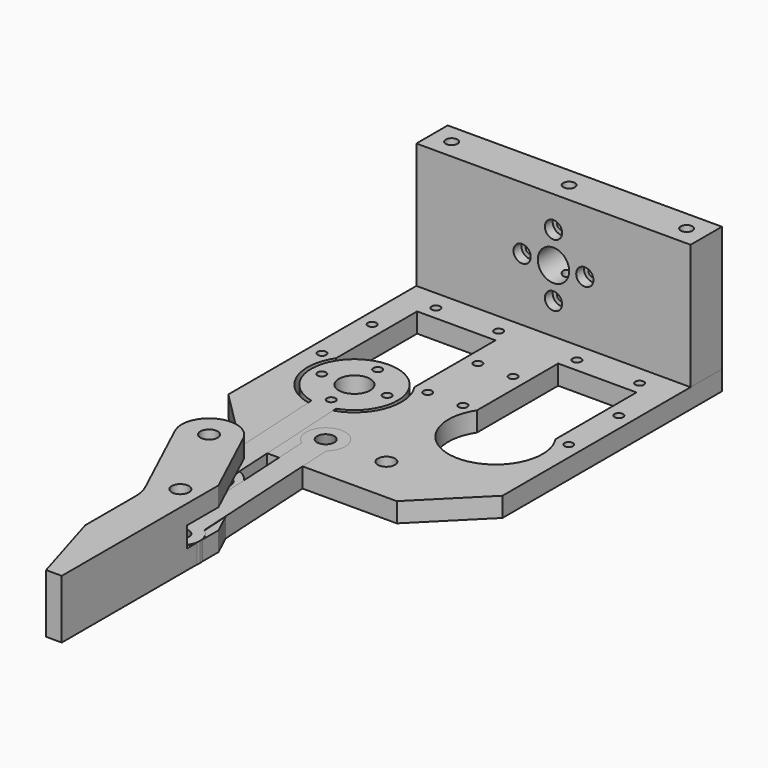
from build123d import *

# Parameters (mm, degrees)
F1_DEPTH        = 5
F2_D            = 2.2
F3_D            = 4.4
F4_D            = 3.3
F5_W            = 70
F5_H            = 10
F5_R            = 1.65
F5_R_2          = 1.5
F6_DEPTH        = 32
F7_R            = 1.1
F7_R_2          = 4
F8_DEPTH        = 10.001
F9_R            = 1.1
F10_DEPTH       = 5
F11_R           = 2.2
F12_DEPTH       = 15
F13_W           = 37
F13_H           = 5.2
F14_DEPTH       = 95.1269579297
F14_DEPTH_BACK  = 38.8526856333
F15_R           = 6.99999
F16_R           = 10
F17_D           = 2.2
F17_CBORE_D     = 4.4
F17_CBORE_DEPTH = 2.5


# Not quite as in the source:
# - a fillet or chamfer is up to 0.001 mm smaller than in the source, because OpenCascade refuses the exact size
# - a feature names something its author has since deleted; it is built from what else it names


with BuildPart() as f1:
    # F0 (on Top) → F1 (new body)
    with BuildSketch(Plane.XY):
        Polygon((0, 0), (15, -15), (55, -15), (70, 0), (70, 70), (0, 70), align=None)
        with BuildLine():
            Line((7, 51.5), (27, 51.5))
            Line((27, 51.5), (27, 25.6332495807))
            ThreePointArc((27, 25.6332495807), (28.4891252931, 22.4641016151), (29, 19))
            ThreePointArc((29, 19), (13.5358983849, 7.5108747069), (7, 25.6332495807))
            Line((7, 25.6332495807), (7, 51.5))
        make_face(mode=Mode.SUBTRACT)
        with BuildLine():
            Line((43, 25.6332495807), (43, 51.5))
            Line((43, 51.5), (63, 51.5))
            Line((63, 51.5), (63, 25.6332495807))
            ThreePointArc((63, 25.6332495807), (64.4891252931, 22.4641016151), (65, 19))
            ThreePointArc((65, 19), (49.5358983849, 7.5108747069), (43, 25.6332495807))
        make_face(mode=Mode.SUBTRACT)
    extrude(amount=F1_DEPTH)

    # F2 (through all)
    with Locations(Plane(origin=(0, 0, 0), x_dir=(1, 0, 0), z_dir=(0, 0, -1))):
        with Locations((9, -55), (3.5, -41.5), (3.5, -25.5), (30.5, -25.5), (30.5, -41.5), (39.5, -25.5), (39.5, -41.5), (66.5, -41.5), (66.5, -25.5), (61, -55), (45, -55), (25, -55)):
            Hole(F2_D / 2)

    # F3 (through all)
    with Locations(Plane(origin=(0, 0, 0), x_dir=(1, 0, 0), z_dir=(0, 0, -1))):
        with Locations((27.2587684794, 3), (42.7412315206, 3)):
            Hole(F3_D / 2)

    # F4 (through all)
    with Locations(Plane(origin=(0, 0, 0), x_dir=(1, 0, 0), z_dir=(0, 0, -1))):
        with Locations((5, -65), (35, -65), (65, -65)):
            Hole(F4_D / 2)


with BuildPart() as f6:
    # F5 (on face) → F6 (new body)
    with BuildSketch(Plane.XY.offset(5)):
        with Locations((35, 65)):
            Rectangle(F5_W, F5_H)
        with Locations((5, 65)):
            Circle(F5_R, mode=Mode.SUBTRACT)
        with Locations((35, 65)):
            Circle(F5_R, mode=Mode.SUBTRACT)
        with Locations((65, 65)):
            Circle(F5_R, mode=Mode.SUBTRACT)
        with Locations((5, 65)):
            Circle(F5_R)
        with Locations((5, 65)):
            Circle(F5_R_2, mode=Mode.SUBTRACT)
        with Locations((35, 65)):
            Circle(F5_R)
        with Locations((35, 65)):
            Circle(F5_R_2, mode=Mode.SUBTRACT)
        with Locations((65, 65)):
            Circle(F5_R)
        with Locations((65, 65)):
            Circle(F5_R_2, mode=Mode.SUBTRACT)
    extrude(amount=F6_DEPTH)

    # F7 (on face) → F8 (cut, through all)
    with BuildSketch(Plane.XZ.offset(-60)):
        with Locations((35, 29)):
            Circle(F7_R)
        with Locations((27, 21)):
            Circle(F7_R)
        with Locations((35, 13)):
            Circle(F7_R)
        with Locations((43, 21)):
            Circle(F7_R)
        with Locations((35, 21)):
            Circle(F7_R_2)
    extrude(amount=-F8_DEPTH, mode=Mode.SUBTRACT)

    # F17 (through all)
    with Locations(Plane.XZ.offset(-60)):
        with Locations((35, 29), (43, 21), (35, 13), (27, 21)):
            CounterBoreHole(F17_D / 2, F17_CBORE_D / 2, F17_CBORE_DEPTH)


with BuildPart() as f10:
    # F9 (on Top) → F10 (new body)
    with BuildSketch(Plane.XY):
        with BuildLine():
            Line((16.8284171456, -31.0896252664), (16.602526778, -27.0960086671))
            ThreePointArc((16.602526778, -27.0960086671), (17.7147808671, -35.4537223569), (24.823629595, -30.9202074907))
            ThreePointArc((24.823629595, -30.9202074907), (24.2308174972, -28.5587048344), (22.5929516769, -26.7571731157))
            Line((22.5929516769, -26.7571731157), (22.8188420445, -30.750789715))
            Line((22.8188420445, -30.750789715), (22.0201187246, -30.7959677885))
            ThreePointArc((22.0201187246, -30.7959677885), (22.0227517023, -30.8580628412), (22.023629595, -30.9202074907))
            ThreePointArc((22.023629595, -30.9202074907), (19.8857742445, -33.1193295979), (17.6271404654, -31.0444471928))
            Line((17.6271404654, -31.0444471928), (16.8284171456, -31.0896252664))
        make_face()
        with BuildLine():
            ThreePointArc((22.5929516769, -26.7571731157), (19.5412666355, -25.9281867416), (16.602526778, -27.0960086671))
            Line((16.602526778, -27.0960086671), (16.8284171456, -31.0896252664))
            Line((16.8284171456, -31.0896252664), (17.6271404654, -31.0444471928))
            ThreePointArc((17.6271404654, -31.0444471928), (19.6993898929, -28.7237183611), (22.0201187246, -30.7959677885))
            Line((22.0201187246, -30.7959677885), (22.8188420445, -30.750789715))
            Line((22.8188420445, -30.750789715), (22.5929516769, -26.7571731157))
        make_face()
        with BuildLine():
            ThreePointArc((20.5928621857, 8.6033014223), (17.6211985109, 8.0175543521), (14.6024372868, 8.2644658709))
            Line((14.6024372868, 8.2644658709), (16.602526778, -27.0960086671))
            ThreePointArc((16.602526778, -27.0960086671), (19.5412666355, -25.9281867416), (22.5929516769, -26.7571731157))
            Line((22.5929516769, -26.7571731157), (20.5928621857, 8.6033014223))
        make_face()
        with BuildLine():
            Line((14.6024372868, 8.2644658709), (14.1541999846, 16.189053136))
            ThreePointArc((14.1541999846, 16.189053136), (15.4806580473, 22.7002162141), (21, 19))
            ThreePointArc((21, 19), (20.7801124014, 17.6920434896), (20.1446248835, 16.5278886874))
            Line((20.1446248835, 16.5278886874), (20.5928621857, 8.6033014223))
            ThreePointArc((20.5928621857, 8.6033014223), (25.9588359747, 12.6172687681), (28, 19))
            ThreePointArc((28, 19), (10.121525963, 27.5840896385), (14.6024372868, 8.2644658709))
        make_face()
        with Locations((9.0127668015, 18.5482192648)):
            Circle(F9_R, mode=Mode.SUBTRACT)
        with Locations((16.5482192648, 26.9872331985)):
            Circle(F9_R, mode=Mode.SUBTRACT)
        with Locations((24.9872331985, 19.4517807352)):
            Circle(F9_R, mode=Mode.SUBTRACT)
        with BuildLine():
            ThreePointArc((20.1446248835, 16.5278886874), (17.2258903676, 15.0063834007), (14.1541999846, 16.189053136))
            Line((14.1541999846, 16.189053136), (14.6024372868, 8.2644658709))
            ThreePointArc((14.6024372868, 8.2644658709), (17.6211985109, 8.0175543521), (20.5928621857, 8.6033014223))
            Line((20.5928621857, 8.6033014223), (20.1446248835, 16.5278886874))
        make_face()
        with Locations((17.4517807352, 11.0127668015)):
            Circle(F9_R, mode=Mode.SUBTRACT)
    extrude(amount=F10_DEPTH)


with BuildPart() as f10b:
    # F9 (on Top) → F10, piece 2 (new body)
    with BuildSketch(Plane.XY):
        with BuildLine():
            ThreePointArc((30.4798712965, -6.8241988236), (27.5411314389, -7.9920207491), (24.4894463976, -7.163034375))
            Line((24.4894463976, -7.163034375), (26.8612952574, -49.0960086671))
            ThreePointArc((26.8612952574, -49.0960086671), (29.8000351149, -47.9281867416), (32.8517201563, -48.7571731157))
            Line((32.8517201563, -48.7571731157), (30.4798712965, -6.8241988236))
        make_face()
        with BuildLine():
            ThreePointArc((30.4798712965, -6.8241988236), (31.7922833457, -5.108848728), (32.2587684794, -3))
            ThreePointArc((32.2587684794, -3), (24.8972658232, 1.4071879021), (24.4894463976, -7.163034375))
            Line((24.4894463976, -7.163034375), (24.26355603, -3.1694177757))
            Line((24.26355603, -3.1694177757), (25.0622793498, -3.1242397022))
            ThreePointArc((25.0622793498, -3.1242397022), (27.1345287772, -0.8035108704), (29.455257609, -2.8757602978))
            Line((29.455257609, -2.8757602978), (30.2539809288, -2.8305822243))
            Line((30.2539809288, -2.8305822243), (30.4798712965, -6.8241988236))
        make_face()
        with BuildLine():
            Line((24.26355603, -3.1694177757), (24.4894463976, -7.163034375))
            ThreePointArc((24.4894463976, -7.163034375), (27.5411314389, -7.9920207491), (30.4798712965, -6.8241988236))
            Line((30.4798712965, -6.8241988236), (30.2539809288, -2.8305822243))
            Line((30.2539809288, -2.8305822243), (29.455257609, -2.8757602978))
            ThreePointArc((29.455257609, -2.8757602978), (29.4578905866, -2.9378553506), (29.4587684794, -3))
            ThreePointArc((29.4587684794, -3), (27.3209131288, -5.1991221072), (25.0622793498, -3.1242397022))
            Line((25.0622793498, -3.1242397022), (24.26355603, -3.1694177757))
        make_face()
        with BuildLine():
            ThreePointArc((32.8517201563, -48.7571731157), (29.8000351149, -47.9281867416), (26.8612952574, -49.0960086671))
            Line((26.8612952574, -49.0960086671), (27.087185625, -53.0896252664))
            Line((27.087185625, -53.0896252664), (27.8859089449, -53.0444471928))
            ThreePointArc((27.8859089449, -53.0444471928), (29.9581583723, -50.7237183611), (32.278887204, -52.7959677885))
            Line((32.278887204, -52.7959677885), (33.0776105239, -52.750789715))
            Line((33.0776105239, -52.750789715), (32.8517201563, -48.7571731157))
        make_face()
        with BuildLine():
            Line((27.087185625, -53.0896252664), (26.8612952574, -49.0960086671))
            ThreePointArc((26.8612952574, -49.0960086671), (27.9735493465, -57.4537223569), (35.0823980744, -52.9202074907))
            ThreePointArc((35.0823980744, -52.9202074907), (34.4895859766, -50.5587048344), (32.8517201563, -48.7571731157))
            Line((32.8517201563, -48.7571731157), (33.0776105239, -52.750789715))
            Line((33.0776105239, -52.750789715), (32.278887204, -52.7959677885))
            ThreePointArc((32.278887204, -52.7959677885), (32.2815201817, -52.8580628412), (32.2823980744, -52.9202074907))
            ThreePointArc((32.2823980744, -52.9202074907), (30.1445427239, -55.1193295979), (27.8859089449, -53.0444471928))
            Line((27.8859089449, -53.0444471928), (27.087185625, -53.0896252664))
        make_face()
    extrude(amount=F10_DEPTH)


with BuildPart() as f12:
    # F11 (on Top) → F12 (new body)
    with BuildSketch(Plane.XY):
        Polygon((35, -96.9026277703), (35, -46.9026277703), (23.2094562721, -21.6177251492), (10.5211472536, -27.5343808136), (25, -58.5843807293), (25, -76.9026277703), (31, -96.9026277703), align=None)
        with Locations((19.823629595, -30.9202074907)):
            Circle(F11_R, mode=Mode.SUBTRACT)
        with Locations((30.0823980744, -52.9202074907)):
            Circle(F11_R, mode=Mode.SUBTRACT)
    extrude(amount=F12_DEPTH)

    # F13 (on face) → F14 (cut, two sides)
    with BuildSketch(Plane(origin=(-1.9042745345, -0.8879777987, 0), x_dir=(0.4226182617, -0.906307787, 0), z_dir=(-0.906307787, -0.4226182617, 0))) as f14_sk:
        with Locations((47.9010527064, 7.5)):
            Rectangle(F13_W, F13_H)
    extrude(amount=-F14_DEPTH, mode=Mode.SUBTRACT)
    extrude(f14_sk.sketch, amount=F14_DEPTH_BACK, mode=Mode.SUBTRACT)

    # F15 (radius 7 in the source; OpenCascade refuses exactly that, so slightly less here)
    f15_edges = [f12.edges().sort_by_distance(p)[0] for p in [
        (10.521147, -27.534381, 12.55),
        (10.521147, -27.534381, 2.45),
        (23.209456, -21.617725, 12.55),
        (23.209456, -21.617725, 2.45),
    ]]
    fillet(f15_edges, radius=F15_R)

    # F16
    f16_edges = [f12.edges().sort_by_distance(p)[0] for p in [
        (25, -58.584381, 12.55),
        (25, -58.584381, 2.45),
    ]]
    fillet(f16_edges, radius=F16_R)


solid = Compound([f1.part, f6.part, f10.part, f10b.part, f12.part])
